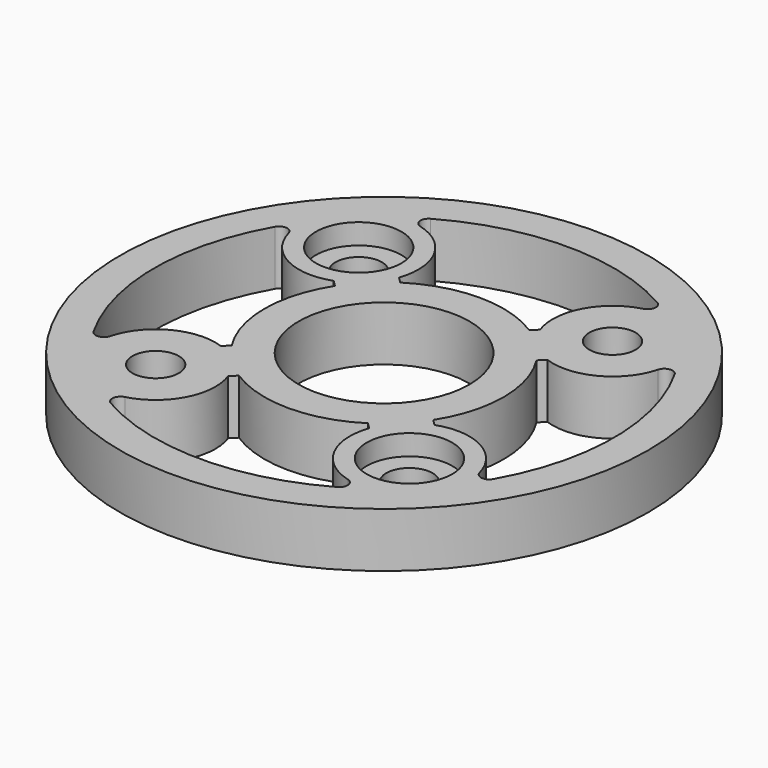
from build123d import *

# Parameters (mm, degrees)
F0_R            = 24.51608
F0_R_2          = 2.15265
F0_R_3          = 7.9375
F1_DEPTH        = 5.08
F3_DEPTH        = 5.08
F3_COPIES_COUNT = 4
F4_R            = 0.762
F5_R            = 3.96875
F6_DEPTH        = 1.905


# Not quite as in the source:
# - a pattern or mirror of a feature is missing from the dataset's text; its kind, count and spacing are read off the source's solid


with BuildPart() as f1:
    # F0 (on Top) → F1 (new body)
    with BuildSketch(Plane.XY):
        Circle(F0_R)
        with Locations((-11.7865906, -11.7865906)):
            Circle(F0_R_2, mode=Mode.SUBTRACT)
        with Locations((11.7865906, -11.7865906)):
            Circle(F0_R_2, mode=Mode.SUBTRACT)
        with Locations((-11.7865906, 11.7865906)):
            Circle(F0_R_2, mode=Mode.SUBTRACT)
        Circle(F0_R_3, mode=Mode.SUBTRACT)
        with Locations((11.7865906, 11.7865906)):
            Circle(F0_R_2, mode=Mode.SUBTRACT)
    extrude(amount=F1_DEPTH)

    # F2 (on face) → F3 (cut, through all)
    with BuildSketch(Plane.XY.offset(5.08)):
        with BuildLine():
            ThreePointArc((-12.5005198818, 17.2967828873), (-7.4612395718, 15.2741760893), (-6.553034663, 9.9206307084))
            Line((-6.553034663, 9.9206307084), (-5.9913991959, 9.3589952413))
            ThreePointArc((-5.9913991959, 9.3589952413), (0, 11.1125), (5.9913991959, 9.3589952413))
            Line((5.9913991959, 9.3589952413), (6.553034663, 9.9206307084))
            ThreePointArc((6.553034663, 9.9206307084), (7.4612395718, 15.2741760893), (12.5005198818, 17.2967828873))
            ThreePointArc((12.5005198818, 17.2967828873), (0, 21.34108), (-12.5005198818, 17.2967828873))
        make_face()
    f3 = extrude(amount=-F3_DEPTH, mode=Mode.SUBTRACT)

    # F3_copies: F3 ×4 about axis
    f3_copies_axis = Axis((0, 0, 0), (0, 0, 1))
    for i in range(1, F3_COPIES_COUNT):
        add(f3.rotate(f3_copies_axis, i * 360 / F3_COPIES_COUNT), mode=Mode.SUBTRACT)

    # F4
    f4_edges = [f1.edges().sort_by_distance(p)[0] for p in [
        (-12.50052, 17.296783, 2.54),
        (12.50052, 17.296783, 2.54),
        (-17.296783, -12.50052, 2.54),
        (-17.296783, 12.50052, 2.54),
        (12.50052, -17.296783, 2.54),
        (-12.50052, -17.296783, 2.54),
        (17.296783, 12.50052, 2.54),
        (17.296783, -12.50052, 2.54),
    ]]
    fillet(f4_edges, radius=F4_R)

    # F5 (on face) → F6 (cut)
    with BuildSketch(Plane.XY.offset(5.08)):
        with Locations((-11.7865906, 11.7865906)):
            Circle(F5_R)
        with Locations((11.7865906, -11.7865906)):
            Circle(F5_R)
    extrude(amount=-F6_DEPTH, mode=Mode.SUBTRACT)


solid = f1.part
